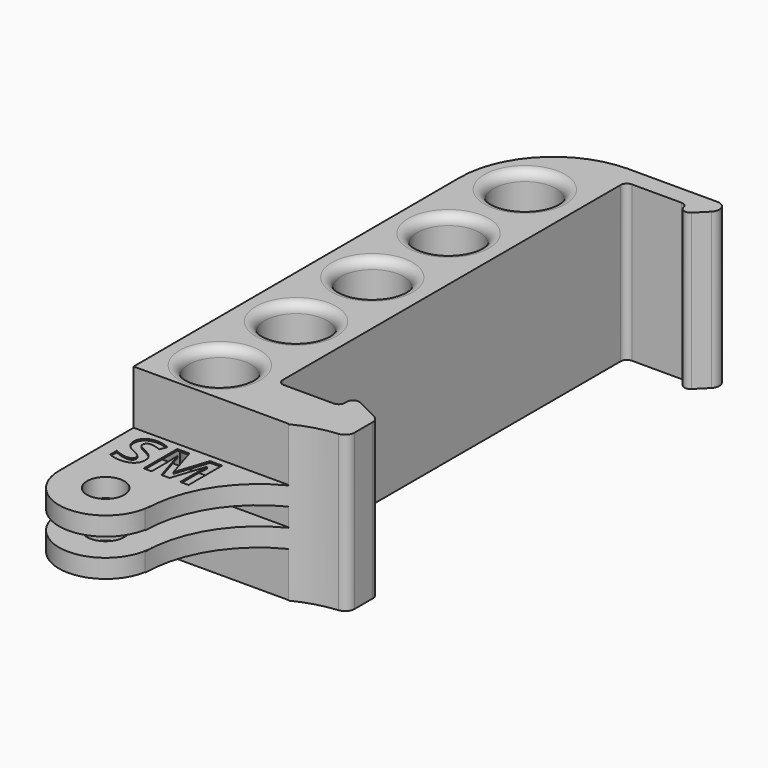
from build123d import *

# Parameters (mm, degrees)
F0_R          = 3
F1_DEPTH      = 25
F2_W          = 15
F2_H          = 7.3227109388
F2_H_2        = 8.6772890612
F2_W_2        = 16.6172117094
F2_H_3        = 3
F3_DEPTH      = 25
F4_R          = 1.5
F5_R          = 1
F6_R          = 5
F7_DEPTH      = 25
F8_R          = 1
F9_R          = 1.5
F10_TEXT_SIZE = 9.479734581
F11_DEPTH     = 0.25


# Not quite as in the source:
# - a feature names something its author has since deleted; it is built from what else it names
# - Text() gives the source's letters only with a copy of the font that has no kerning and outlines rounded to 1/6400 em; it was checked with that copy


with BuildPart() as f1:
    # F0 (on Top) → F1 (new body)
    with BuildSketch(Plane.XY):
        with BuildLine():
            Line((-6.9643953955, 0), (-6.9643953955, 70))
            Line((-6.9643953955, 70), (3.0356046045, 70))
            Line((3.0356046045, 70), (3.0356046045, 67))
            Line((3.0356046045, 67), (9.0356046045, 73))
            Line((9.0356046045, 73), (-8.9999945524, 73))
            ThreePointArc((-8.9999945524, 73), (-19.6316873132, 68.549217828), (-24.0162145794, 57.890030544))
            Line((-24.0162145794, 57.890030544), (-23.8977254927, -7.8553749621))
            Line((-23.8977254927, -7.8553749621), (-23.8977254927, -22.8553749621))
            ThreePointArc((-23.8977254927, -22.8553749621), (-16.3977254927, -30.3553749621), (-8.8977254927, -22.8553749621))
            Line((-8.8977254927, -22.8553749621), (-8.8977254927, -24.264943873))
            ThreePointArc((-8.8977254927, -24.264943873), (-3.664939404, -11.4663843539), (9.0356046045, -6))
            Line((9.0356046045, -6), (9.0356046045, 0))
            Line((9.0356046045, 0), (3.0356046045, 3))
            Line((3.0356046045, 3), (3.0356046045, 0))
            Line((3.0356046045, 0), (-6.9643953955, 0))
        make_face()
        with Locations((-16.3977254927, -22.8553749621)):
            Circle(F0_R, mode=Mode.SUBTRACT)
    extrude(amount=F1_DEPTH)

    # F2 (on face) → F3 (cut)
    with BuildSketch(Plane(origin=(-23.8977254927, 0, 0), x_dir=(0, -1, 0), z_dir=(-1, 0, 0))):
        with Locations((15.3553749621, 3.6613554694)):
            Rectangle(F2_W, F2_H)
        with Locations((15.3553749621, 20.6613554694)):
            Rectangle(F2_W, F2_H_2)
        Polygon((39.6337285638, 7.3227109388), (22.8553749621, 7.3227109388), (22.8553749621, 0), (7.8553749621, 0), (7.8553749621, -18.6784230173), (39.6337285638, -18.6784230173), align=None)
        Polygon((22.8553749621, 25), (22.8553749621, 16.3227109388), (39.6337285638, 16.3227109388), (39.6337285638, 38.9752238989), (7.8553749621, 38.9752238989), (7.8553749621, 25), align=None)
        with Locations((31.1639808168, 11.8227109388)):
            Rectangle(F2_W_2, F2_H_3)
        with Locations((15.3553749621, 11.8227109388)):
            Rectangle(F2_W, F2_H_3)
    extrude(amount=-F3_DEPTH, mode=Mode.SUBTRACT)

    # F4
    f4_edges = [f1.edges().sort_by_distance(p)[0] for p in [
        (9.035605, 0, 12.5),
        (9.035605, -6, 12.5),
        (9.035605, 73, 12.5),
    ]]
    fillet(f4_edges, radius=F4_R)

    # F5
    f5_edges = [f1.edges().sort_by_distance(p)[0] for p in [
        (-6.964395, 70, 12.5),
        (-6.964395, 0, 12.5),
        (3.035605, 70, 12.5),
        (3.035605, 0, 12.5),
    ]]
    fillet(f5_edges, radius=F5_R)

    # F6 (on face) → F7 (cut)
    with BuildSketch(Plane.XY.offset(25)):
        with Locations((-15.6192537578, 60.5245295457)):
            Circle(F6_R)
        with Locations((-15.6226723807, 45.1834524206)):
            Circle(F6_R)
        with Locations((-15.6295096266, 14.5012981705)):
            Circle(F6_R)
        with Locations((-15.6329282495, -0.8397789546)):
            Circle(F6_R)
        with Locations((-15.6260910036, 29.8423752956)):
            Circle(F6_R)
    extrude(amount=-F7_DEPTH, mode=Mode.SUBTRACT)

    # F8
    f8_edges = [f1.edges().sort_by_distance(p)[0] for p in [
        (3.035605, 67, 12.5),
        (3.035605, 3, 12.5),
    ]]
    fillet(f8_edges, radius=F8_R)

    # F9
    f9_edges = [f1.edges().sort_by_distance(p)[0] for p in [
        (-20.619254, 60.52453, 25),
        (-20.622672, 45.183452, 25),
        (-20.626091, 29.842375, 25),
        (-20.62951, 14.501298, 25),
        (-20.632928, -0.839779, 25),
    ]]
    fillet(f9_edges, radius=F9_R)

    # F10 (on face) → F11 (cut)
    with BuildSketch(Plane.XY.offset(16.3227109388)):
        with Locations((-22.0727809152, -15.7146737841)):
            Text('SM', F10_TEXT_SIZE, font='Open Sans', font_style=FontStyle.BOLD, text_align=(TextAlign.LEFT, TextAlign.BOTTOM))
    extrude(amount=-F11_DEPTH, mode=Mode.SUBTRACT)


solid = f1.part
